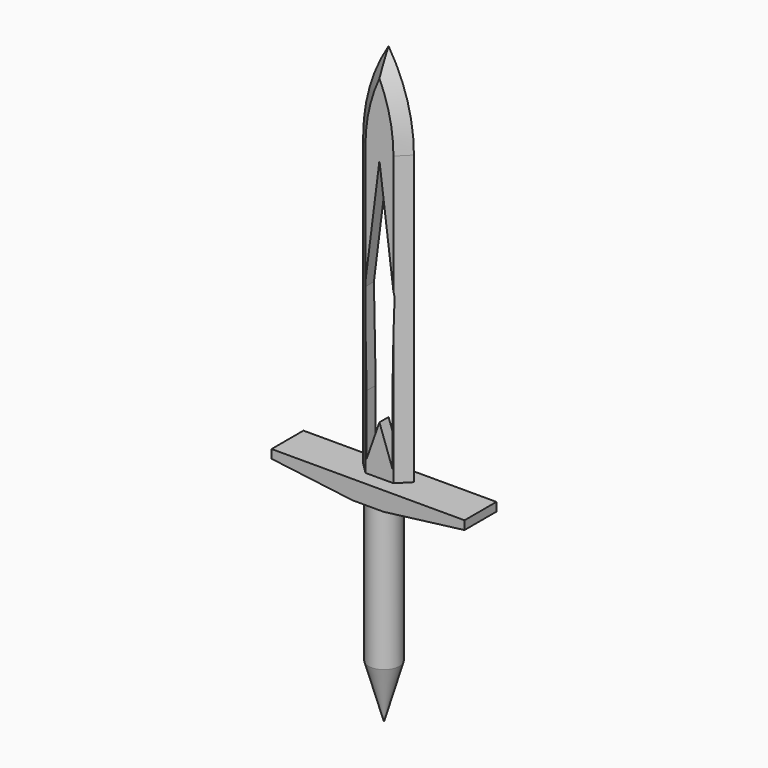
from build123d import *

# Parameters (mm, degrees)
F0_W        = 6.9019780494
F0_H        = 64.2322748899
F3_DEPTH    = 8.89
F4_DEPTH    = 2.54
F5_T1_DEPTH = 141.4955107475
F5_T4_ANGLE = 42.5345423557
F5_T6_ANGLE = 42.5345423557


# Not quite as in the source:
# - a fillet or chamfer that OpenCascade refuses, or shapes differently, is made with other operations: its cross-section is extruded or revolved along the edge and cut away or added


with BuildPart() as f1:
    # F0 (on Front) → F1 (revolve)
    with BuildSketch(Plane.XZ):
        with Locations((3.4509890247, -32.116137445)):
            Rectangle(F0_W, F0_H)
    revolve(axis=Axis((0, 0, -32.116137445), (0, 0, -1)))

    # F0 (on Front) → F2 (revolve)
    with BuildSketch(Plane.XZ):
        Polygon((6.9019780494, -64.2322748899), (0, -64.2322748899), (0, -88.3597657084), align=None)
    revolve(axis=Axis((0, 0, -76.2960202992), (0, 0, 1)))


with BuildPart() as f3:
    # F0 (on Front) → F3 (new body, symmetric)
    with BuildSketch(Plane.XZ):
        Polygon((-43.0214107037, 4.5587546192), (-6.9019780494, 0), (0, 0), (6.9019780494, 0), (43.0214107037, 4.5587546192), (43.0214107037, 8.4022246301), (11.3210510463, 8.4022246301), (0, 8.4022246301), (-11.3210510463, 8.4022246301), (-43.0214107037, 8.4022246301), align=None)
    extrude(amount=F3_DEPTH, both=True)


with BuildPart() as f4:
    # F0 (on Front) → F4 (new body, symmetric)
    with BuildSketch(Plane.XZ):
        with BuildLine():
            Line((-11.3210510463, 136.8335857987), (-11.3210510463, 8.4022246301))
            Line((-11.3210510463, 8.4022246301), (0, 8.4022246301))
            Line((0, 8.4022246301), (11.3210510463, 8.4022246301))
            Line((11.3210510463, 8.4022246301), (11.3210510463, 136.8335857987))
            ThreePointArc((11.3210510463, 136.8335857987), (8.4338116967, 157.1828142535), (0, 175.9257614613))
            ThreePointArc((0, 175.9257614613), (-8.4338116967, 157.1828142535), (-11.3210510463, 136.8335857987))
        make_face()
        Polygon((-5.7232712246, 40.8455764441), (-6.5300096758, 81.3025683165), (0, 133.073836565), (6.5300096758, 81.3025683165), (5.7232712246, 40.8455764441), (5.7232712246, 14.0499221161), (0, 30.3084515035), (-5.7232712246, 14.0499221161), align=None, mode=Mode.SUBTRACT)
    extrude(amount=F4_DEPTH, both=True)

    # F5: chamfer of 5.08 on 2 edges, made by hand

    # F5_s2 → F5_t1 (cut)
    with BuildSketch(Plane.XY.offset(-4.6619249487)):
        Polygon((-11.3210510463, 2.54), (-6.2410510463, -2.54), (-11.3210510463, -2.54), align=None)
        Polygon((11.3210510463, 2.54), (6.2410510463, -2.54), (11.3210510463, -2.54), align=None)
    extrude(amount=F5_T1_DEPTH, mode=Mode.SUBTRACT)

    # F5_s3 → F5_t4 (revolve, cut)
    with BuildSketch(Plane.XY.offset(136.8335857987)):
        Polygon((11.3210510463, 2.54), (6.2410510463, -2.54), (11.3210510463, -2.54), align=None)
    revolve(axis=Axis((-61.8331281927, -2.54, 136.8335857987), (0, -1, 0)), revolution_arc=F5_T4_ANGLE, mode=Mode.SUBTRACT)

    # F5_s5 → F5_t6 (revolve, cut)
    with BuildSketch(Plane(origin=(96.4227325292, 0, 105.0996687872), x_dir=(0, 1, 0), z_dir=(0.676034573, 0, 0.7368699045))):
        Polygon((2.54, 120.0954427185), (-2.54, 115.0154427185), (-2.54, 120.0954427185), align=None)
    revolve(axis=Axis((61.8331281927, -2.54, 136.8335857987), (0, -1, 0)), revolution_arc=F5_T6_ANGLE, mode=Mode.SUBTRACT)


solid = Compound([f1.part, f3.part, f4.part])
